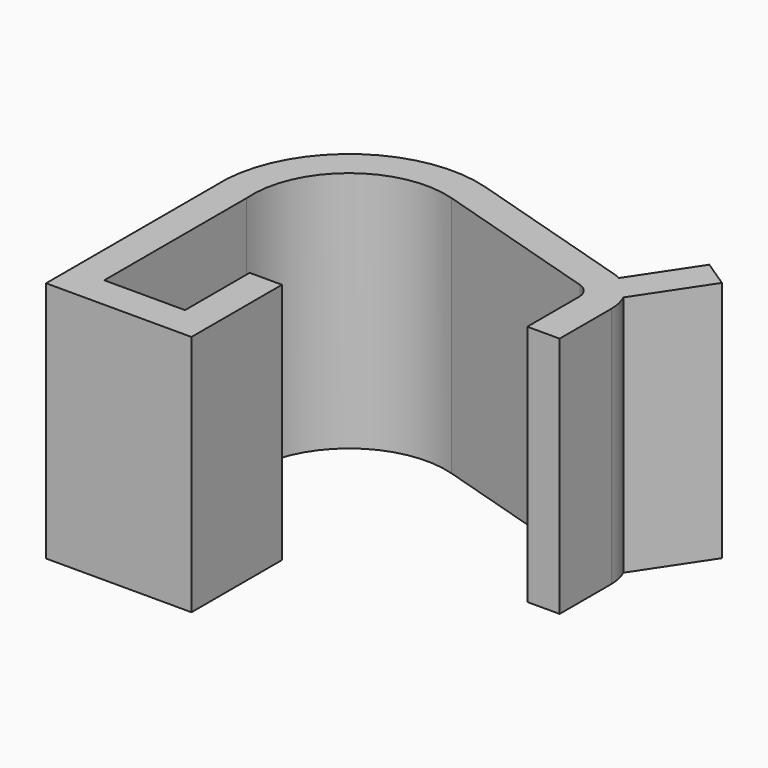
from build123d import *

# Parameters (mm, degrees)
F0_W     = 2
F0_H     = 4
F1_DEPTH = 15
F2_W     = 2
F2_H     = 4
F3_DEPTH = 15


# Not quite as in the source:
# - a feature names something its author has since deleted; it is built from what else it names


with BuildPart() as f1:
    # F0 (on Top) → F1 (new body)
    with BuildSketch(Plane.XY):
        with BuildLine():
            Line((7, 32.0000030547), (2, 32.0000030547))
            Line((2, 32.0000030547), (2, 43.0000030547))
            ThreePointArc((2, 43.0000030547), (4.22965477, 48.1459058579), (9.7375987459, 49.20147642))
            Line((9.7375987459, 49.20147642), (10.3227891625, 51.113949211))
            ThreePointArc((10.3227891625, 51.113949211), (3.4424209582, 50.0513163902), (0, 44.0000030547))
            Line((0, 44.0000030547), (0, 30.0000030547))
            Line((0, 30.0000030547), (9, 30.0000030547))
            Line((9, 30.0000030547), (9, 37.0000030547))
            Line((9, 37.0000030547), (7, 37.0000030547))
            Line((7, 37.0000030547), (7, 32.0000030547))
        make_face()
        Polygon((10.3227891625, 51.113949211), (9.7375987459, 49.20147642), (20.2561990964, 45.9829291287), (20.841389513, 47.8954019197), align=None)
        with BuildLine():
            Line((20.841389513, 47.8954019197), (20.2561990964, 45.9829291287))
            ThreePointArc((20.2561990964, 45.9829291287), (20.7938383415, 45.6028219427), (21, 44.9774941877))
            Line((21, 44.9774941877), (23, 44.9774941877))
            ThreePointArc((23, 44.9774941877), (22.9273260191, 45.6394915882), (22.7127657141, 46.2699564496))
            ThreePointArc((22.7127657141, 46.2699564496), (22.1205825647, 47.1207678466), (21.277739528, 47.7242382529))
            ThreePointArc((21.277739528, 47.7242382529), (21.0628558439, 47.8182107047), (20.841389513, 47.8954019197))
        make_face()
        with Locations((22, 42.9774941877)):
            Rectangle(F0_W, F0_H)
        with BuildLine():
            Line((23.8132360697, 51.5414804224), (21.277739528, 47.7242382529))
            ThreePointArc((21.277739528, 47.7242382529), (22.1205825647, 47.1207678466), (22.7127657141, 46.2699564496))
            Line((22.7127657141, 46.2699564496), (25.4792139424, 50.4349011311))
            Line((25.4792139424, 50.4349011311), (23.8132360697, 51.5414804224))
        make_face()
    extrude(amount=F1_DEPTH)


with BuildPart() as f3:
    # F2 (on Top) → F3 (new body)
    with BuildSketch(Plane.XY):
        with Locations((-37.8, -36.9225088671)):
            Rectangle(F2_W, F2_H)
        with BuildLine():
            ThreePointArc((-39.5438009036, -33.9170739261), (-39.0061616585, -34.2971811121), (-38.8, -34.9225088671))
            Line((-38.8, -34.9225088671), (-36.8, -34.9225088671))
            ThreePointArc((-36.8, -34.9225088671), (-36.8726739809, -34.2605114665), (-37.0872342859, -33.6300466052))
            ThreePointArc((-37.0872342859, -33.6300466052), (-37.6794174353, -32.7792352081), (-38.522260472, -32.1757648018))
            ThreePointArc((-38.522260472, -32.1757648018), (-38.7371441561, -32.0817923501), (-38.958610487, -32.0046011351))
            Line((-38.958610487, -32.0046011351), (-39.5438009036, -33.9170739261))
        make_face()
        Polygon((-50.0624012541, -30.6985266348), (-39.5438009036, -33.9170739261), (-38.958610487, -32.0046011351), (-49.4772108375, -28.7860538438), align=None)
        with BuildLine():
            ThreePointArc((-57.8, -36.9), (-55.57034523, -31.7540971969), (-50.0624012541, -30.6985266348))
            Line((-50.0624012541, -30.6985266348), (-49.4772108375, -28.7860538438))
            ThreePointArc((-49.4772108375, -28.7860538438), (-56.3575790418, -29.8486866645), (-59.8, -35.9))
            Line((-59.8, -35.9), (-59.8, -49.9))
            Line((-59.8, -49.9), (-50.8, -49.9))
            Line((-50.8, -49.9), (-50.8, -42.9))
            Line((-50.8, -42.9), (-52.8, -42.9))
            Line((-52.8, -42.9), (-52.8, -47.9))
            Line((-52.8, -47.9), (-57.8, -47.9))
            Line((-57.8, -47.9), (-57.8, -36.9))
        make_face()
        with BuildLine():
            ThreePointArc((-38.522260472, -32.1757648018), (-37.6794174353, -32.7792352081), (-37.0872342859, -33.6300466052))
            Line((-37.0872342859, -33.6300466052), (-34.3207860576, -29.4651019236))
            Line((-34.3207860576, -29.4651019236), (-35.9867639303, -28.3585226323))
            Line((-35.9867639303, -28.3585226323), (-38.522260472, -32.1757648018))
        make_face()
    extrude(amount=F3_DEPTH)


with BuildPart() as f3b:
    # F2 (on Top) → F3, piece 2 (new body)
    with BuildSketch(Plane.XY):
        with Locations((33.034186706, 0.0025241677)):
            Rectangle(F2_W, F2_H)
        with BuildLine():
            ThreePointArc((31.2903858024, 3.0079591087), (31.8280250475, 2.6278519227), (32.034186706, 2.0025241677))
            Line((32.034186706, 2.0025241677), (34.034186706, 2.0025241677))
            ThreePointArc((34.034186706, 2.0025241677), (33.9615127251, 2.6645215683), (33.7469524201, 3.2949864296))
            ThreePointArc((33.7469524201, 3.2949864296), (33.1547692707, 4.1457978267), (32.311926234, 4.749268233))
            ThreePointArc((32.311926234, 4.749268233), (32.0970425499, 4.8432406847), (31.875576219, 4.9204318997))
            Line((31.875576219, 4.9204318997), (31.2903858024, 3.0079591087))
        make_face()
        Polygon((20.7717854519, 6.2265064), (31.2903858024, 3.0079591087), (31.875576219, 4.9204318997), (21.3569758685, 8.138979191), align=None)
        with BuildLine():
            ThreePointArc((13.034186706, 0.0250330348), (15.2638414761, 5.1709358379), (20.7717854519, 6.2265064))
            Line((20.7717854519, 6.2265064), (21.3569758685, 8.138979191))
            ThreePointArc((21.3569758685, 8.138979191), (14.4766076642, 7.0763463703), (11.034186706, 1.0250330348))
            Line((11.034186706, 1.0250330348), (11.034186706, -12.9749669652))
            Line((11.034186706, -12.9749669652), (20.034186706, -12.9749669652))
            Line((20.034186706, -12.9749669652), (20.034186706, -5.9749669652))
            Line((20.034186706, -5.9749669652), (18.034186706, -5.9749669652))
            Line((18.034186706, -5.9749669652), (18.034186706, -10.9749669652))
            Line((18.034186706, -10.9749669652), (13.034186706, -10.9749669652))
            Line((13.034186706, -10.9749669652), (13.034186706, 0.0250330348))
        make_face()
        with BuildLine():
            ThreePointArc((32.311926234, 4.749268233), (33.1547692707, 4.1457978267), (33.7469524201, 3.2949864296))
            Line((33.7469524201, 3.2949864296), (36.5134006484, 7.4599311112))
            Line((36.5134006484, 7.4599311112), (34.8474227758, 8.5665104025))
            Line((34.8474227758, 8.5665104025), (32.311926234, 4.749268233))
        make_face()
    extrude(amount=F3_DEPTH)


with BuildPart() as f3c:
    # F2 (on Top) → F3, piece 3 (new body)
    with BuildSketch(Plane.XY):
        with Locations((-12.8, -36.9225088671)):
            Rectangle(F2_W, F2_H)
        with BuildLine():
            ThreePointArc((-14.5438009036, -33.9170739261), (-14.0061616585, -34.2971811121), (-13.8, -34.9225088671))
            Line((-13.8, -34.9225088671), (-11.8, -34.9225088671))
            ThreePointArc((-11.8, -34.9225088671), (-11.8726739809, -34.2605114665), (-12.0872342859, -33.6300466052))
            ThreePointArc((-12.0872342859, -33.6300466052), (-12.6794174353, -32.7792352081), (-13.522260472, -32.1757648018))
            ThreePointArc((-13.522260472, -32.1757648018), (-13.7371441561, -32.0817923501), (-13.958610487, -32.0046011351))
            Line((-13.958610487, -32.0046011351), (-14.5438009036, -33.9170739261))
        make_face()
        Polygon((-25.0624012541, -30.6985266348), (-14.5438009036, -33.9170739261), (-13.958610487, -32.0046011351), (-24.4772108375, -28.7860538438), align=None)
        with BuildLine():
            ThreePointArc((-32.8, -36.9), (-30.57034523, -31.7540971969), (-25.0624012541, -30.6985266348))
            Line((-25.0624012541, -30.6985266348), (-24.4772108375, -28.7860538438))
            ThreePointArc((-24.4772108375, -28.7860538438), (-31.3575790418, -29.8486866645), (-34.8, -35.9))
            Line((-34.8, -35.9), (-34.8, -49.9))
            Line((-34.8, -49.9), (-25.8, -49.9))
            Line((-25.8, -49.9), (-25.8, -42.9))
            Line((-25.8, -42.9), (-27.8, -42.9))
            Line((-27.8, -42.9), (-27.8, -47.9))
            Line((-27.8, -47.9), (-32.8, -47.9))
            Line((-32.8, -47.9), (-32.8, -36.9))
        make_face()
        with BuildLine():
            ThreePointArc((-13.522260472, -32.1757648018), (-12.6794174353, -32.7792352081), (-12.0872342859, -33.6300466052))
            Line((-12.0872342859, -33.6300466052), (-9.3207860576, -29.4651019236))
            Line((-9.3207860576, -29.4651019236), (-10.9867639303, -28.3585226323))
            Line((-10.9867639303, -28.3585226323), (-13.522260472, -32.1757648018))
        make_face()
    extrude(amount=F3_DEPTH)


with BuildPart() as f3d:
    # F2 (on Top) → F3, piece 4 (new body)
    with BuildSketch(Plane.XY):
        with Locations((58.034186706, 0.0025241677)):
            Rectangle(F2_W, F2_H)
        with BuildLine():
            ThreePointArc((56.2903858024, 3.0079591087), (56.8280250475, 2.6278519227), (57.034186706, 2.0025241677))
            Line((57.034186706, 2.0025241677), (59.034186706, 2.0025241677))
            ThreePointArc((59.034186706, 2.0025241677), (58.9615127251, 2.6645215683), (58.7469524201, 3.2949864296))
            ThreePointArc((58.7469524201, 3.2949864296), (58.1547692707, 4.1457978267), (57.311926234, 4.749268233))
            ThreePointArc((57.311926234, 4.749268233), (57.0970425499, 4.8432406847), (56.875576219, 4.9204318997))
            Line((56.875576219, 4.9204318997), (56.2903858024, 3.0079591087))
        make_face()
        Polygon((45.7717854519, 6.2265064), (56.2903858024, 3.0079591087), (56.875576219, 4.9204318997), (46.3569758685, 8.138979191), align=None)
        with BuildLine():
            ThreePointArc((38.034186706, 0.0250330348), (40.2638414761, 5.1709358379), (45.7717854519, 6.2265064))
            Line((45.7717854519, 6.2265064), (46.3569758685, 8.138979191))
            ThreePointArc((46.3569758685, 8.138979191), (39.4766076642, 7.0763463703), (36.034186706, 1.0250330348))
            Line((36.034186706, 1.0250330348), (36.034186706, -12.9749669652))
            Line((36.034186706, -12.9749669652), (45.034186706, -12.9749669652))
            Line((45.034186706, -12.9749669652), (45.034186706, -5.9749669652))
            Line((45.034186706, -5.9749669652), (43.034186706, -5.9749669652))
            Line((43.034186706, -5.9749669652), (43.034186706, -10.9749669652))
            Line((43.034186706, -10.9749669652), (38.034186706, -10.9749669652))
            Line((38.034186706, -10.9749669652), (38.034186706, 0.0250330348))
        make_face()
        with BuildLine():
            ThreePointArc((57.311926234, 4.749268233), (58.1547692707, 4.1457978267), (58.7469524201, 3.2949864296))
            Line((58.7469524201, 3.2949864296), (61.5134006484, 7.4599311112))
            Line((61.5134006484, 7.4599311112), (59.8474227758, 8.5665104025))
            Line((59.8474227758, 8.5665104025), (57.311926234, 4.749268233))
        make_face()
    extrude(amount=F3_DEPTH)


with BuildPart() as f3e:
    # F2 (on Top) → F3, piece 5 (new body)
    with BuildSketch(Plane.XY):
        with Locations((12.2, -36.9225088671)):
            Rectangle(F2_W, F2_H)
        with BuildLine():
            ThreePointArc((10.4561990964, -33.9170739261), (10.9938383415, -34.2971811121), (11.2, -34.9225088671))
            Line((11.2, -34.9225088671), (13.2, -34.9225088671))
            ThreePointArc((13.2, -34.9225088671), (13.1273260191, -34.2605114665), (12.9127657141, -33.6300466052))
            ThreePointArc((12.9127657141, -33.6300466052), (12.3205825647, -32.7792352081), (11.477739528, -32.1757648018))
            ThreePointArc((11.477739528, -32.1757648018), (11.2628558439, -32.0817923501), (11.041389513, -32.0046011351))
            Line((11.041389513, -32.0046011351), (10.4561990964, -33.9170739261))
        make_face()
        Polygon((-0.0624012541, -30.6985266348), (10.4561990964, -33.9170739261), (11.041389513, -32.0046011351), (0.5227891625, -28.7860538438), align=None)
        with BuildLine():
            ThreePointArc((-7.8, -36.9), (-5.57034523, -31.7540971969), (-0.0624012541, -30.6985266348))
            Line((-0.0624012541, -30.6985266348), (0.5227891625, -28.7860538438))
            ThreePointArc((0.5227891625, -28.7860538438), (-6.3575790418, -29.8486866645), (-9.8, -35.9))
            Line((-9.8, -35.9), (-9.8, -49.9))
            Line((-9.8, -49.9), (-0.8, -49.9))
            Line((-0.8, -49.9), (-0.8, -42.9))
            Line((-0.8, -42.9), (-2.8, -42.9))
            Line((-2.8, -42.9), (-2.8, -47.9))
            Line((-2.8, -47.9), (-7.8, -47.9))
            Line((-7.8, -47.9), (-7.8, -36.9))
        make_face()
        with BuildLine():
            ThreePointArc((11.477739528, -32.1757648018), (12.3205825647, -32.7792352081), (12.9127657141, -33.6300466052))
            Line((12.9127657141, -33.6300466052), (15.6792139424, -29.4651019236))
            Line((15.6792139424, -29.4651019236), (14.0132360697, -28.3585226323))
            Line((14.0132360697, -28.3585226323), (11.477739528, -32.1757648018))
        make_face()
    extrude(amount=F3_DEPTH)


with BuildPart() as f1_1:
    # F5: moved
    add(f1.part.moved(Location((-10.3, -40.1, 0))))


solid = f1_1.part
